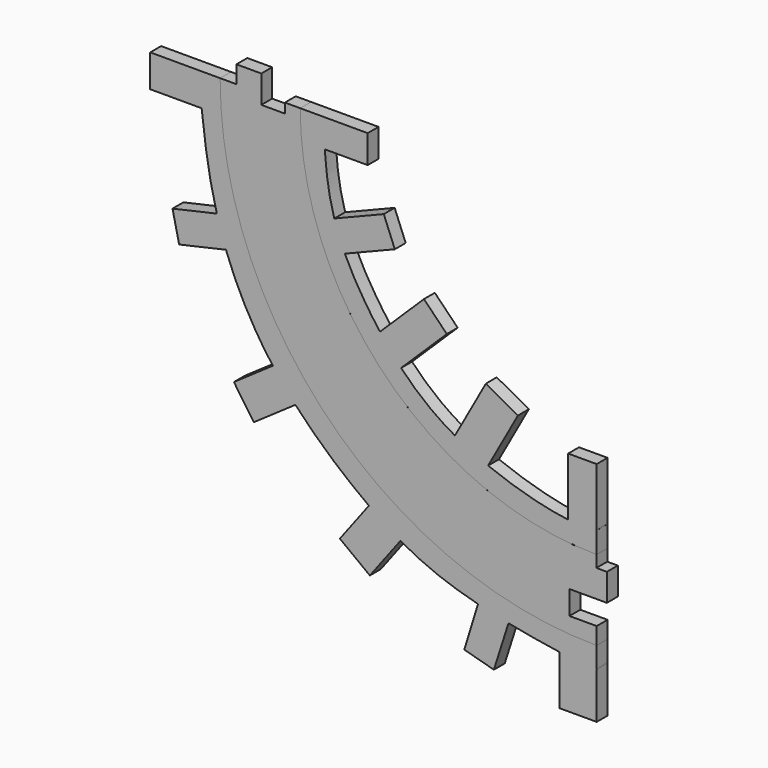
from build123d import *

# Parameters (mm, degrees)
F1_DEPTH = 3.175
F3_DEPTH = 3.175


# Not quite as in the source:
# - ends of sketch curves that miss each other by under 0.0002 mm in the source are joined


with BuildPart() as f1:
    # F0 (on Front) → F1 (new body)
    with BuildSketch(Plane.XZ):
        with BuildLine():
            ThreePointArc((-4.57723355, -43.7883980573), (-66.819423743, -17.9873487673), (-92.5539227851, 44.2823866067))
            Line((-92.5539227851, 44.2823866067), (-97.6339227851, 44.2823866067))
            add(Edge.make_bspline(
                [(-97.6339227851, 44.2823866067), (-97.3931684107, 41.7497203339), (-97.1524140363, 39.2170540611), (-96.8805696251, 36.6884975094)],
                knots=[0, 0, 0, 0, 0.0522468531, 0.0522468531, 0.0522468531, 0.0522468531], degree=3))
            add(Edge.make_bspline(
                [(-96.8805696251, 36.6884975094), (-96.1391179528, 29.7918963404), (-95.1663820006, 22.9258681136), (-93.3315372634, 16.1738000838)],
                knots=[0.0522468531, 0.0522468531, 0.0522468531, 0.0522468531, 0.194749384, 0.194749384, 0.194749384, 0.194749384], degree=3))
            add(Edge.make_bspline(
                [(-93.3315372634, 16.1738000838), (-92.7163937389, 13.910125757), (-92.0043518732, 11.6592602013), (-91.1919757647, 9.4312911762)],
                knots=[0.194749384, 0.194749384, 0.194749384, 0.194749384, 0.242524276, 0.242524276, 0.242524276, 0.242524276], degree=3))
            add(Edge.make_bspline(
                [(-91.1919757647, 9.4312911762), (-88.6009408677, 2.3252901097), (-84.9892452149, -4.5477935635), (-80.2454108338, -10.8606620469)],
                knots=[0.242524276, 0.242524276, 0.242524276, 0.242524276, 0.394900018, 0.394900018, 0.394900018, 0.394900018], degree=3))
            add(Edge.make_bspline(
                [(-80.2454108338, -10.8606620469), (-78.607242384, -13.0406584688), (-76.8340664871, -15.1538492769), (-74.9712769181, -17.1861090489)],
                knots=[0.394900018, 0.394900018, 0.394900018, 0.394900018, 0.4475192945, 0.4475192945, 0.4475192945, 0.4475192945], degree=3))
            add(Edge.make_bspline(
                [(-74.9712769181, -17.1861090489), (-69.6272612199, -23.016304958), (-63.5457113797, -28.1804261391), (-57.7984134089, -32.3449592406)],
                knots=[0.4475192945, 0.4475192945, 0.4475192945, 0.4475192945, 0.5984747456, 0.5984747456, 0.5984747456, 0.5984747456], degree=3))
            add(Edge.make_bspline(
                [(-57.7984134089, -32.3449592406), (-55.3415292823, -34.1252350021), (-52.9457275098, -35.7228425466), (-50.4258841879, -37.168898271)],
                knots=[0.5984747456, 0.5984747456, 0.5984747456, 0.5984747456, 0.6630059486, 0.6630059486, 0.6630059486, 0.6630059486], degree=3))
            add(Edge.make_bspline(
                [(-50.4258841879, -37.168898271), (-45.3798949167, -40.0646265916), (-39.8364976619, -42.3526304388), (-32.3091378654, -44.2827760941)],
                knots=[0.6630059486, 0.6630059486, 0.6630059486, 0.6630059486, 0.7922297598, 0.7922297598, 0.7922297598, 0.7922297598], degree=3))
            add(Edge.make_bspline(
                [(-32.3091378654, -44.2827760941), (-30.0596561185, -44.8595822437), (-27.6329950376, -45.4044295862), (-25.1835874199, -45.9026667789)],
                knots=[0.7922297598, 0.7922297598, 0.7922297598, 0.7922297598, 0.8308470987, 0.8308470987, 0.8308470987, 0.8308470987], degree=3))
            add(Edge.make_bspline(
                [(-25.1835874199, -45.9026667789), (-21.0258896893, -46.7483894877), (-16.802653084, -47.4598158509), (-13.2691699484, -47.9652898008)],
                knots=[0.8308470987, 0.8308470987, 0.8308470987, 0.8308470987, 0.8963973245, 0.8963973245, 0.8963973245, 0.8963973245], degree=3))
            add(Edge.make_bspline(
                [(-13.2691699484, -47.9652898008), (-8.4519136222, -48.6544108435), (-4.916655331, -48.9607420913), (-4.57723355, -48.70271393)],
                knots=[0.8963973245, 0.8963973245, 0.8963973245, 0.8963973245, 0.9857630376, 0.9857630376, 0.9857630376, 0.9857630376], degree=3))
            Line((-4.57723355, -48.70271393), (-4.57723355, -48.5507466091))
            Line((-4.57723355, -48.5507466091), (-4.57723355, -43.7883980573))
        make_face()
        with BuildLine():
            add(Edge.make_bspline(
                [(-97.6339227851, 44.2823866067), (-97.3931684107, 41.7497203339), (-97.1524140363, 39.2170540611), (-96.8805696251, 36.6884975094)],
                knots=[0, 0, 0, 0, 0.0522468531, 0.0522468531, 0.0522468531, 0.0522468531], degree=3))
            Line((-97.6339227851, 44.2823866067), (-108.8849874868, 44.2823866067))
            Line((-108.8849874868, 44.2823866067), (-108.8849874868, 36.6884975094))
            Line((-108.8849874868, 36.6884975094), (-96.8805696251, 36.6884975094))
        make_face()
        with BuildLine():
            add(Edge.make_bspline(
                [(-4.57723355, -48.70271393), (-4.5231598458, -48.6616071441), (-4.5501966979, -48.6061768766), (-4.57723355, -48.5507466091)],
                knots=[0.9857630376, 0.9857630376, 0.9857630376, 0.9857630376, 1, 1, 1, 1], degree=3))
            Line((-4.57723355, -48.5507466091), (-4.57723355, -48.70271393))
        make_face()
        with BuildLine():
            Line((-4.57723355, -59.5153173973), (-4.57723355, -48.70271393))
            add(Edge.make_bspline(
                [(-13.2691699484, -47.9652898008), (-8.4519136222, -48.6544108435), (-4.916655331, -48.9607420913), (-4.57723355, -48.70271393)],
                knots=[0.8963973245, 0.8963973245, 0.8963973245, 0.8963973245, 0.9857630376, 0.9857630376, 0.9857630376, 0.9857630376], degree=3))
            Line((-13.2691699484, -47.9652898008), (-13.2691699484, -59.5153173973))
            Line((-13.2691699484, -59.5153173973), (-4.57723355, -59.5153173973))
        make_face()
        with BuildLine():
            add(Edge.make_bspline(
                [(-93.3315372634, 16.1738000838), (-92.7163937389, 13.910125757), (-92.0043518732, 11.6592602013), (-91.1919757647, 9.4312911762)],
                knots=[0.194749384, 0.194749384, 0.194749384, 0.194749384, 0.242524276, 0.242524276, 0.242524276, 0.242524276], degree=3))
            Line((-93.3315372634, 16.1738000838), (-103.6843064573, 13.8317355646))
            Line((-103.6843064573, 13.8317355646), (-102.1290715587, 6.9570368465))
            Line((-102.1290715587, 6.9570368465), (-91.1919757647, 9.4312911762))
        make_face()
        with BuildLine():
            Line((-28.5986802118, -56.592917115), (-25.1835874199, -45.9026667789))
            add(Edge.make_bspline(
                [(-32.3091378654, -44.2827760941), (-30.0596561185, -44.8595822437), (-27.6329950376, -45.4044295862), (-25.1835874199, -45.9026667789)],
                knots=[0.7922297598, 0.7922297598, 0.7922297598, 0.7922297598, 0.8308470987, 0.8308470987, 0.8308470987, 0.8308470987], degree=3))
            Line((-32.3091378654, -44.2827760941), (-35.5125362565, -54.710556085))
            Line((-35.5125362565, -54.710556085), (-28.5986802118, -56.592917115))
        make_face()
        with BuildLine():
            add(Edge.make_bspline(
                [(-80.2454108338, -10.8606620469), (-78.607242384, -13.0406584688), (-76.8340664871, -15.1538492769), (-74.9712769181, -17.1861090489)],
                knots=[0.394900018, 0.394900018, 0.394900018, 0.394900018, 0.4475192945, 0.4475192945, 0.4475192945, 0.4475192945], degree=3))
            Line((-80.2454108338, -10.8606620469), (-89.3403956863, -17.1692187548))
            Line((-89.3403956863, -17.1692187548), (-84.6648700593, -23.9098785797))
            Line((-84.6648700593, -23.9098785797), (-74.9712769181, -17.1861090489))
        make_face()
        with BuildLine():
            Line((-57.5702740184, -46.6306970593), (-50.4258841879, -37.168898271))
            add(Edge.make_bspline(
                [(-57.7984134089, -32.3449592406), (-55.3415292823, -34.1252350021), (-52.9457275098, -35.7228425466), (-50.4258841879, -37.168898271)],
                knots=[0.5984747456, 0.5984747456, 0.5984747456, 0.5984747456, 0.6630059486, 0.6630059486, 0.6630059486, 0.6630059486], degree=3))
            Line((-57.7984134089, -32.3449592406), (-64.5855489224, -41.3336219678))
            Line((-64.5855489224, -41.3336219678), (-57.5702740184, -46.6306970593))
        make_face()
    extrude(amount=F1_DEPTH)


with BuildPart() as f1b:
    # F0 (on Front) → F1, piece 2 (new body)
    with BuildSketch(Plane.XZ):
        with BuildLine():
            Line((-68.460035245, 44.188341444), (-73.8470553452, 44.188341444))
            ThreePointArc((-73.8470553452, 44.188341444), (-53.5583942729, -4.792819279), (-4.57723355, -25.0814803512))
            Line((-4.57723355, -25.0814803512), (-4.57723355, -20.089340043))
            add(Edge.make_bspline(
                [(-11.2417986909, -20.089340043), (-7.6185165541, -20.5216548463), (-4.8185609122, -20.3880627705), (-4.57723355, -20.089340043)],
                knots=[0.8679520206, 0.8679520206, 0.8679520206, 0.8679520206, 0.9836335446, 0.9836335446, 0.9836335446, 0.9836335446], degree=3))
            add(Edge.make_bspline(
                [(-29.9419627206, -15.043763619), (-23.422756241, -17.6607776775), (-16.4738824823, -19.4650697847), (-11.2417986909, -20.089340043)],
                knots=[0.7009058442, 0.7009058442, 0.7009058442, 0.7009058442, 0.8679520206, 0.8679520206, 0.8679520206, 0.8679520206], degree=3))
            add(Edge.make_bspline(
                [(-37.6919303949, -11.3869210218), (-35.2854498907, -12.7286211423), (-32.6507981172, -13.9563520855), (-29.9419627206, -15.043763619)],
                knots=[0.6314954647, 0.6314954647, 0.6314954647, 0.6314954647, 0.7009058442, 0.7009058442, 0.7009058442, 0.7009058442], degree=3))
            add(Edge.make_bspline(
                [(-50.2679967336, -1.5694799865), (-46.7502062379, -5.2841732571), (-42.7188946441, -8.5842062158), (-37.6919303949, -11.3869210218)],
                knots=[0.486502187, 0.486502187, 0.486502187, 0.486502187, 0.6314954647, 0.6314954647, 0.6314954647, 0.6314954647], degree=3))
            add(Edge.make_bspline(
                [(-55.2009748713, 4.2784686576), (-53.6443043314, 2.2331240714), (-52.019825963, 0.2804051212), (-50.2679967336, -1.5694799865)],
                knots=[0.4142967892, 0.4142967892, 0.4142967892, 0.4142967892, 0.486502187, 0.486502187, 0.486502187, 0.486502187], degree=3))
            add(Edge.make_bspline(
                [(-63.4136220682, 17.660311036), (-61.2402617068, 12.9621183463), (-58.3602666711, 8.429533519), (-55.2009748713, 4.2784686576)],
                knots=[0.2677545922, 0.2677545922, 0.2677545922, 0.2677545922, 0.4142967892, 0.4142967892, 0.4142967892, 0.4142967892], degree=3))
            add(Edge.make_bspline(
                [(-65.8834584942, 24.0971257956), (-65.2299828846, 21.9310450164), (-64.3936435193, 19.7788412618), (-63.4136220682, 17.660311036)],
                knots=[0.2016751241, 0.2016751241, 0.2016751241, 0.2016751241, 0.2677545922, 0.2677545922, 0.2677545922, 0.2677545922], degree=3))
            add(Edge.make_bspline(
                [(-68.1166645486, 37.6055160739), (-67.7985284224, 33.0703711751), (-67.2281449465, 28.5543686299), (-65.8834584942, 24.0971257956)],
                knots=[0.0657004003, 0.0657004003, 0.0657004003, 0.0657004003, 0.2016751241, 0.2016751241, 0.2016751241, 0.2016751241], degree=3))
            add(Edge.make_bspline(
                [(-68.460035245, 44.188341444), (-68.3652085595, 41.992576638), (-68.270381874, 39.7968118321), (-68.1166645486, 37.6055160739)],
                knots=[0, 0, 0, 0, 0.0657004003, 0.0657004003, 0.0657004003, 0.0657004003], degree=3))
        make_face()
        with BuildLine():
            Line((-58.0849874868, 44.188341444), (-68.460035245, 44.188341444))
            add(Edge.make_bspline(
                [(-68.460035245, 44.188341444), (-68.3652085595, 41.992576638), (-68.270381874, 39.7968118321), (-68.1166645486, 37.6055160739)],
                knots=[0, 0, 0, 0, 0.0657004003, 0.0657004003, 0.0657004003, 0.0657004003], degree=3))
            Line((-68.1166645486, 37.6055160739), (-58.0849874868, 37.6055160739))
            Line((-58.0849874868, 37.6055160739), (-58.0849874868, 44.188341444))
        make_face()
        with BuildLine():
            add(Edge.make_bspline(
                [(-11.2417986909, -20.089340043), (-7.6185165541, -20.5216548463), (-4.8185609122, -20.3880627705), (-4.57723355, -20.089340043)],
                knots=[0.8679520206, 0.8679520206, 0.8679520206, 0.8679520206, 0.9836335446, 0.9836335446, 0.9836335446, 0.9836335446], degree=3))
            Line((-4.57723355, -20.089340043), (-4.57723355, -19.9559408889))
            Line((-4.57723355, -19.9559408889), (-4.57723355, -6.4825667786))
            Line((-4.57723355, -6.4825667786), (-11.2417986909, -6.4825667786))
            Line((-11.2417986909, -6.4825667786), (-11.2417986909, -20.089340043))
        make_face()
        with BuildLine():
            Line((-4.57723355, -19.9559408889), (-4.57723355, -20.089340043))
            add(Edge.make_bspline(
                [(-4.57723355, -20.089340043), (-4.5430909024, -20.0470771818), (-4.5601622262, -20.0015090354), (-4.57723355, -19.9559408889)],
                knots=[0.9836335446, 0.9836335446, 0.9836335446, 0.9836335446, 1, 1, 1, 1], degree=3))
        make_face()
        with BuildLine():
            Line((-54.3195477878, 28.7565803399), (-65.8834584942, 24.0971257956))
            add(Edge.make_bspline(
                [(-65.8834584942, 24.0971257956), (-65.2299828846, 21.9310450164), (-64.3936435193, 19.7788412618), (-63.4136220682, 17.660311036)],
                knots=[0.2016751241, 0.2016751241, 0.2016751241, 0.2016751241, 0.2677545922, 0.2677545922, 0.2677545922, 0.2677545922], degree=3))
            Line((-63.4136220682, 17.660311036), (-51.7432430301, 22.3626649389))
            Line((-51.7432430301, 22.3626649389), (-54.3195477878, 28.7565803399))
        make_face()
        with BuildLine():
            add(Edge.make_bspline(
                [(-37.6919303949, -11.3869210218), (-35.2854498907, -12.7286211423), (-32.6507981172, -13.9563520855), (-29.9419627206, -15.043763619)],
                knots=[0.6314954647, 0.6314954647, 0.6314954647, 0.6314954647, 0.7009058442, 0.7009058442, 0.7009058442, 0.7009058442], degree=3))
            Line((-29.9419627206, -15.043763619), (-22.9809752827, -2.4805746691))
            Line((-22.9809752827, -2.4805746691), (-30.460795653, 1.6638297367))
            Line((-30.460795653, 1.6638297367), (-37.6919303949, -11.3869210218))
        make_face()
        with BuildLine():
            Line((-44.9346528444, 14.3355632134), (-55.2009748713, 4.2784686576))
            add(Edge.make_bspline(
                [(-55.2009748713, 4.2784686576), (-53.6443043314, 2.2331240714), (-52.019825963, 0.2804051212), (-50.2679967336, -1.5694799865)],
                knots=[0.4142967892, 0.4142967892, 0.4142967892, 0.4142967892, 0.486502187, 0.486502187, 0.486502187, 0.486502187], degree=3))
            Line((-50.2679967336, -1.5694799865), (-39.5955882998, 8.8854249421))
            Line((-39.5955882998, 8.8854249421), (-44.9346528444, 14.3355632134))
        make_face()
    extrude(amount=F1_DEPTH)


with BuildPart() as f3:
    # F2 (on Front) → F3 (new body)
    with BuildSketch(Plane.XZ):
        with BuildLine():
            Line((-88.7539610267, 44.2823866067), (-92.5539227851, 44.2823866067))
            ThreePointArc((-92.5539227851, 44.2823866067), (-66.819423743, -17.9873487673), (-4.57723355, -43.7883980573))
            Line((-4.57723355, -43.7883980573), (-4.57723355, -39.7976860404))
            Line((-4.57723355, -39.7976860404), (-10.9395096079, -39.7976860404))
            Line((-10.9395096079, -39.7976860404), (-10.9395096079, -34.2512689531))
            Line((-10.9395096079, -34.2512689531), (-2.193643013, -34.2512689531))
            Line((-2.193643013, -34.2512689531), (-2.193643013, -27.864491567))
            Line((-2.193643013, -27.864491567), (-4.6415692195, -27.864491567))
            Line((-4.6415692195, -27.864491567), (-4.6415692195, -25.0813551247))
            ThreePointArc((-4.6415692195, -25.0813551247), (-53.5811351193, -4.7700678696), (-73.8470553452, 44.188341444))
            Line((-73.8470553452, 44.188341444), (-77.4248614907, 44.188341444))
            Line((-77.4248614907, 44.188341444), (-77.4248614907, 41.9153422117))
            Line((-77.4248614907, 41.9153422117), (-82.9305946827, 41.9153422117))
            Line((-82.9305946827, 41.9153422117), (-82.9305946827, 48.3739897609))
            Line((-82.9305946827, 48.3739897609), (-88.7539610267, 48.3739897609))
            Line((-88.7539610267, 48.3739897609), (-88.7539610267, 44.2823866067))
        make_face()
    extrude(amount=F3_DEPTH)


solid = Compound([f1.part, f1b.part, f3.part])
